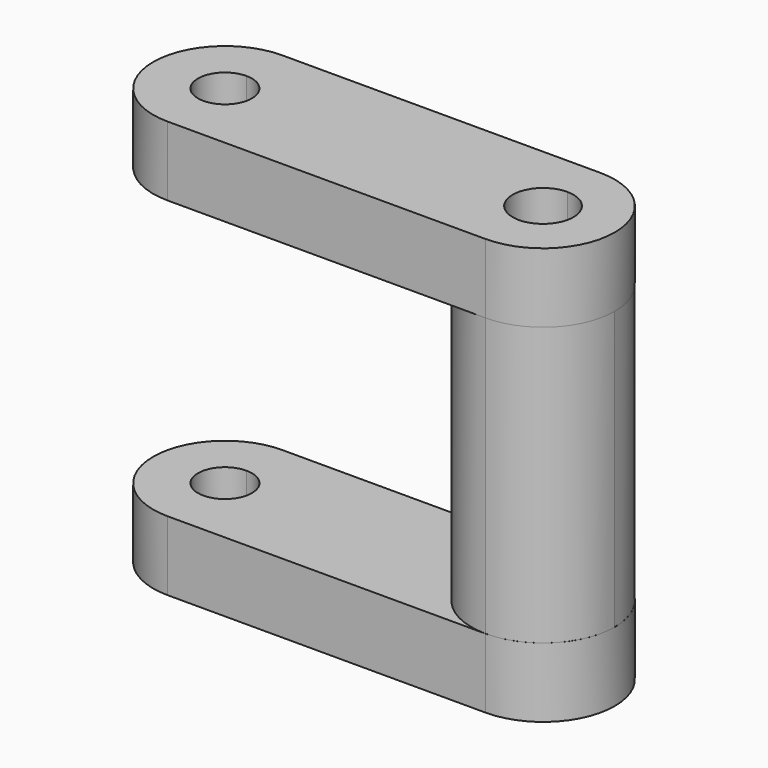
from build123d import *

# Parameters (mm, degrees)
F1_DEPTH = 76.2
F2_DEPTH = 25.4


with BuildPart() as f1:
    # F0 (on Top) → F1 (new body)
    with BuildSketch(Plane.XY):
        with BuildLine():
            ThreePointArc((58.131363, 26.186049), (31.945314, 0), (58.131363, -26.186049))
            Line((58.131363, -26.186049), (58.131363, -11.104064))
            ThreePointArc((58.131363, -11.104064), (47.027299, 0), (58.131363, 11.104064))
            Line((58.131363, 11.104064), (58.131363, 26.186049))
        make_face()
        with BuildLine():
            Line((58.131363, -11.104064), (58.131363, -26.186049))
            ThreePointArc((58.131363, -26.186049), (76.647696, -18.516333), (84.317412, 0))
            ThreePointArc((84.317412, 0), (76.647696, 18.516333), (58.131363, 26.186049))
            Line((58.131363, 26.186049), (58.131363, 11.104064))
            ThreePointArc((58.131363, 11.104064), (65.983122, 7.851759), (69.235427, 0))
            ThreePointArc((69.235427, 0), (65.983122, -7.851759), (58.131363, -11.104064))
        make_face()
    extrude(amount=F1_DEPTH)

    # F0 (on Top) → F2 (join)
    with BuildSketch(Plane.XY):
        with BuildLine():
            Line((-58.131363, -26.208181), (58.131363, -26.208181))
            Line((58.131363, -26.208181), (58.131363, -26.186049))
            ThreePointArc((58.131363, -26.186049), (31.945314, 0), (58.131363, 26.186049))
            Line((58.131363, 26.186049), (58.131363, 26.208181))
            Line((58.131363, 26.208181), (-58.131363, 26.208181))
            Line((-58.131363, 26.208181), (-58.131363, 9.857005))
            ThreePointArc((-58.131363, 9.857005), (-51.161408, 6.969955), (-48.274358, 0))
            ThreePointArc((-48.274358, 0), (-51.161408, -6.969955), (-58.131363, -9.857005))
            Line((-58.131363, -9.857005), (-58.131363, -26.208181))
        make_face()
        with BuildLine():
            Line((58.131363, -26.186049), (58.131363, -26.208181))
            ThreePointArc((58.131363, -26.208181), (84.339544, 0), (58.131363, 26.208181))
            Line((58.131363, 26.208181), (58.131363, 26.186049))
            ThreePointArc((58.131363, 26.186049), (76.647696, 18.516333), (84.317412, 0))
            ThreePointArc((84.317412, 0), (76.647696, -18.516333), (58.131363, -26.186049))
        make_face()
        with BuildLine():
            ThreePointArc((-58.131363, 26.208181), (-84.339544, 0), (-58.131363, -26.208181))
            Line((-58.131363, -26.208181), (-58.131363, -9.857005))
            ThreePointArc((-58.131363, -9.857005), (-67.988368, 0), (-58.131363, 9.857005))
            Line((-58.131363, 9.857005), (-58.131363, 26.208181))
        make_face()
    extrude(amount=F2_DEPTH)

    # F3: F1 across face


with BuildPart() as f1_1:
    add(f1.part)
    add(f1.part.mirror(Plane(origin=(58.131363, 0, 76.2), x_dir=(1, 0, 0), z_dir=(0, 0, 1))))


solid = f1_1.part
